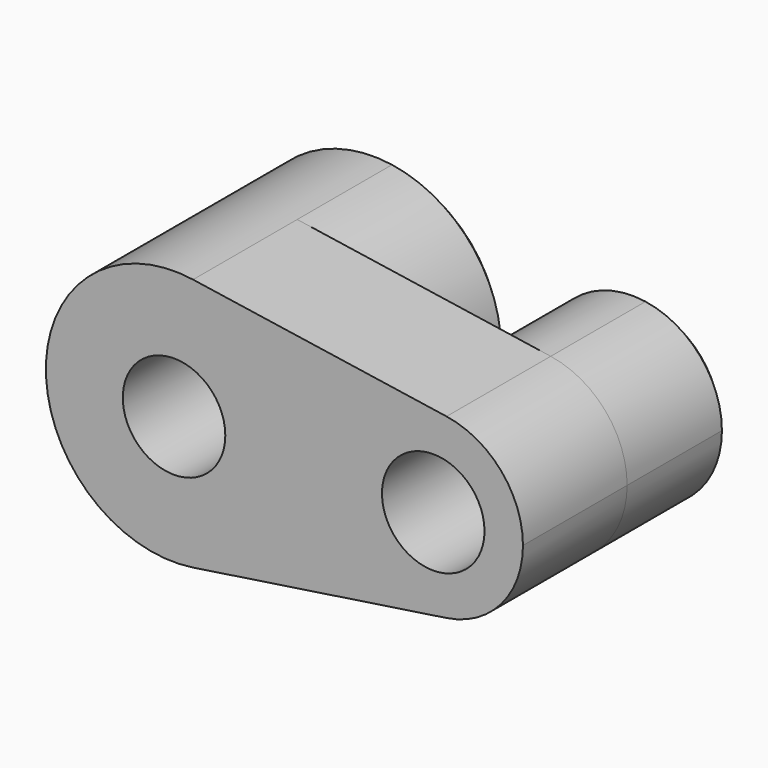
from build123d import *

# Parameters (mm, degrees)
F0_R     = 10
F1_DEPTH = 25.4
F3_DEPTH = 25.4
F4_DEPTH = 25.4
F5_SIZE  = 2.286


# Not quite as in the source:
# - the program builds the solid bodies; features that only make, move or delete a surface that nothing else refers to are left out


with BuildPart() as f1:
    # F0 (on Front) → F1 (new body)
    with BuildSketch(Plane.XZ):
        with BuildLine():
            ThreePointArc((3.7085113233, -24.7234088217), (18.9435052601, -16.313908436), (25, 0))
            ThreePointArc((25, 0), (18.9435052601, 16.313908436), (3.7085113233, 24.7234088217))
            ThreePointArc((3.7085113233, 24.7234088217), (-25, 0), (3.7085113233, -24.7234088217))
        make_face()
        Circle(F0_R, mode=Mode.SUBTRACT)
        with BuildLine():
            ThreePointArc((3.7085113233, 24.7234088217), (18.9435052601, 16.313908436), (25, 0))
            ThreePointArc((25, 0), (18.9435052601, -16.313908436), (3.7085113233, -24.7234088217))
            Line((3.7085113233, -24.7234088217), (53.1553289667, -17.3063861752))
            ThreePointArc((53.1553289667, -17.3063861752), (33.0593710404, 0), (53.1553289667, 17.3063861752))
            Line((53.1553289667, 17.3063861752), (3.7085113233, 24.7234088217))
        make_face()
        with BuildLine():
            ThreePointArc((68.0593710404, 0), (63.8198247225, 11.4197359052), (53.1553289667, 17.3063861752))
            ThreePointArc((53.1553289667, 17.3063861752), (33.0593710404, 0), (53.1553289667, -17.3063861752))
            ThreePointArc((53.1553289667, -17.3063861752), (63.8198247225, -11.4197359052), (68.0593710404, 0))
        make_face()
        with Locations((50.5593710404, 0)):
            Circle(F0_R, mode=Mode.SUBTRACT)
    extrude(amount=F1_DEPTH)

    # F0 (on Front) → F3 (join)
    with BuildSketch(Plane.XZ):
        with BuildLine():
            ThreePointArc((3.7085113233, -24.7234088217), (18.9435052601, -16.313908436), (25, 0))
            ThreePointArc((25, 0), (18.9435052601, 16.313908436), (3.7085113233, 24.7234088217))
            ThreePointArc((3.7085113233, 24.7234088217), (-25, 0), (3.7085113233, -24.7234088217))
        make_face()
        Circle(F0_R, mode=Mode.SUBTRACT)
        with BuildLine():
            ThreePointArc((68.0593710404, 0), (63.8198247225, 11.4197359052), (53.1553289667, 17.3063861752))
            ThreePointArc((53.1553289667, 17.3063861752), (33.0593710404, 0), (53.1553289667, -17.3063861752))
            ThreePointArc((53.1553289667, -17.3063861752), (63.8198247225, -11.4197359052), (68.0593710404, 0))
        make_face()
        with Locations((50.5593710404, 0)):
            Circle(F0_R, mode=Mode.SUBTRACT)
    extrude(amount=F3_DEPTH)

    # F0 (on Front) → F4 (join)
    with BuildSketch(Plane.XZ):
        with BuildLine():
            ThreePointArc((3.7085113233, -24.7234088217), (18.9435052601, -16.313908436), (25, 0))
            ThreePointArc((25, 0), (18.9435052601, 16.313908436), (3.7085113233, 24.7234088217))
            ThreePointArc((3.7085113233, 24.7234088217), (-25, 0), (3.7085113233, -24.7234088217))
        make_face()
        Circle(F0_R, mode=Mode.SUBTRACT)
        with BuildLine():
            ThreePointArc((68.0593710404, 0), (63.8198247225, 11.4197359052), (53.1553289667, 17.3063861752))
            ThreePointArc((53.1553289667, 17.3063861752), (33.0593710404, 0), (53.1553289667, -17.3063861752))
            ThreePointArc((53.1553289667, -17.3063861752), (63.8198247225, -11.4197359052), (68.0593710404, 0))
        make_face()
        with Locations((50.5593710404, 0)):
            Circle(F0_R, mode=Mode.SUBTRACT)
    extrude(amount=-F4_DEPTH)

    # F5
    f5_edges = [f1.edges().sort_by_distance(p)[0] for p in [
        (-10, 25.4, 0),
        (-25, 25.4, 0),
        (33.059371, 25.4, 0),
        (40.559371, 25.4, 0),
    ]]
    chamfer(f5_edges, length=F5_SIZE)


solid = f1.part
